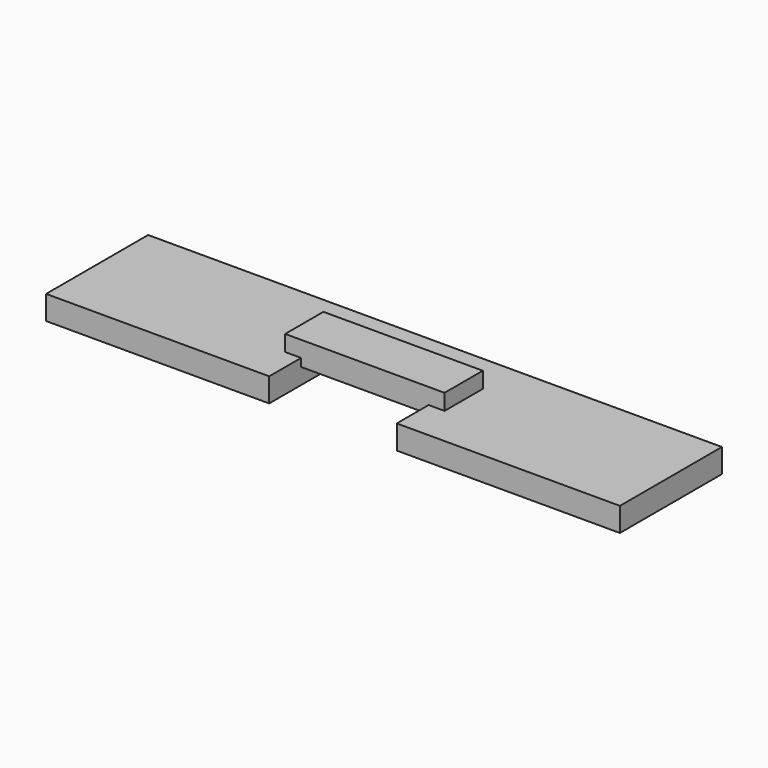
from build123d import *

# Parameters (mm, degrees)
F0_W      = 57.15
F0_H      = 12.7
F1_DEPTH  = 2.38125
F2_W      = 15.875
F2_H      = 4.7625
F3_DEPTH  = 1.5875
F5_W      = 12.7
F5_H      = 4.7625
F6_DEPTH  = 3.175
F7_W      = 12.7
F7_H      = 3.96875
F8_DEPTH  = 2.38225
F9_W      = 12.7
F9_H      = 2
F10_DEPTH = 2.38225
F11_W     = 12.7
F11_H     = 4.7625
F12_DEPTH = 1.5875


# Not quite as in the source:
# - a feature of the source that left no trace in its solid (it failed there, or was rolled back) is left out
# - a length typed as a fraction of an inch, garbled in the dataset ("3 / 203.2 mm" for 3/8 in), is restored


with BuildPart() as f1:
    # F0 (on Top) → F1 (new body)
    with BuildSketch(Plane.XY):
        Rectangle(F0_W, F0_H)
    extrude(amount=F1_DEPTH)

    # F2 (on face) → F3 (join)
    with BuildSketch(Plane.XY.offset(2.38125)):
        Rectangle(F2_W, F2_H)
    extrude(amount=F3_DEPTH)

    # F5 (on offset) → F6 (cut, through all)
    with BuildSketch(Plane.XY.offset(3.175)):
        Rectangle(F5_W, F5_H)
    extrude(amount=-F6_DEPTH, mode=Mode.SUBTRACT)

    # F7 (on face) → F8 (cut, through all)
    with BuildSketch(Plane.XY.offset(2.38125)):
        with Locations((0, -4.365625)):
            Rectangle(F7_W, F7_H)
    extrude(amount=-F8_DEPTH, mode=Mode.SUBTRACT)

    # F9 (on face) → F10 (cut, through all)
    with BuildSketch(Plane.XY.offset(2.38125)):
        with Locations((0, 3.38125)):
            Rectangle(F9_W, F9_H)
    extrude(amount=-F10_DEPTH, mode=Mode.SUBTRACT)

    # F11 (on face) → F12 (join)
    with BuildSketch(Plane(origin=(0, 0, 3.175), x_dir=(1, 0, 0), z_dir=(0, 0, -1))):
        Rectangle(F11_W, F11_H)
    extrude(amount=F12_DEPTH)


solid = f1.part
